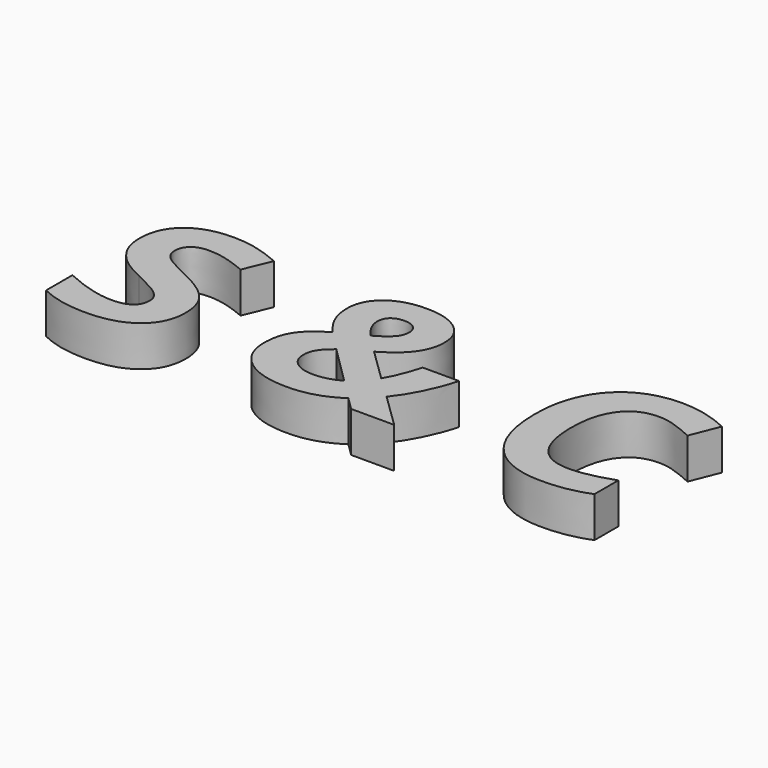
from build123d import *

# Parameters (mm, degrees)
F0_TEXT_SIZE = 14.6554989947
F1_DEPTH     = 2.54


# Not quite as in the source:
# - Text() gives the source's letters only with a copy of the font that has no kerning and outlines rounded to 1/6400 em; it was checked with that copy


with BuildPart() as f1:
    # F0 (on Top) → F1 (new body)
    with BuildSketch(Plane.XY):
        with Locations((63.8279989362, 66.1881268024)):
            Text('S & C', F0_TEXT_SIZE, font='Open Sans', font_style=FontStyle.BOLD, text_align=(TextAlign.LEFT, TextAlign.BOTTOM))
    extrude(amount=F1_DEPTH)


solid = f1.part
